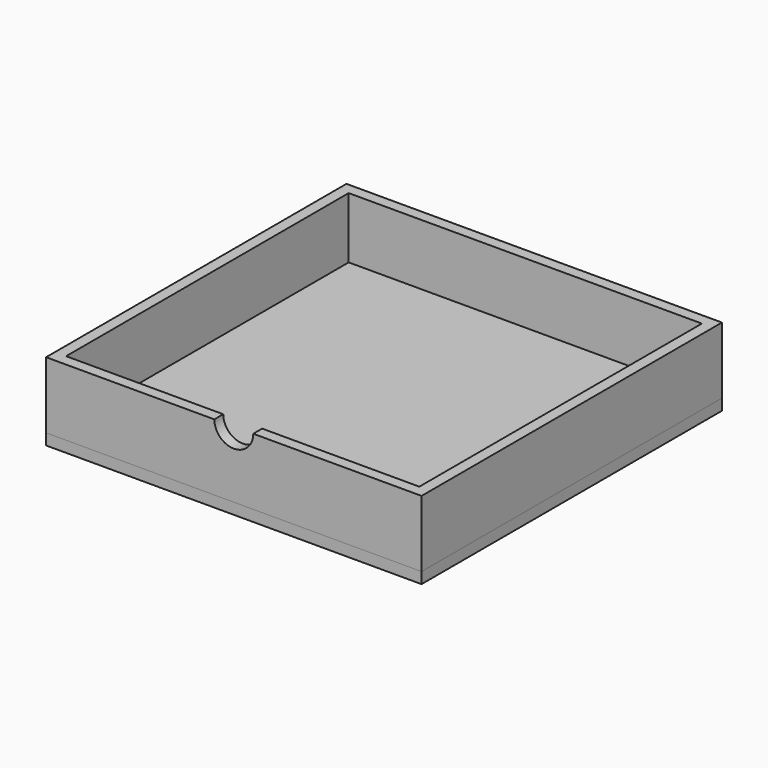
from build123d import *

# Parameters (mm, degrees)
F0_W     = 67.5
F0_H     = 67.5
F0_W_2   = 63.5
F0_H_2   = 63.5
F0_R     = 3.5
F1_DEPTH = 3
F2_DEPTH = 13.97
F4_DEPTH = 2
F5_DEPTH = 2
F6_DEPTH = 3


with BuildPart() as f1:
    # F0 (on Top) → F1 (new body)
    with BuildSketch(Plane.XY):
        Rectangle(F0_W, F0_H)
        Rectangle(F0_W_2, F0_H_2, mode=Mode.SUBTRACT)
        Rectangle(F0_W_2, F0_H_2)
        Circle(F0_R, mode=Mode.SUBTRACT)
    extrude(amount=F1_DEPTH)

    # F0 (on Top) → F2 (join)
    with BuildSketch(Plane.XY):
        Rectangle(F0_W, F0_H)
        Rectangle(F0_W_2, F0_H_2, mode=Mode.SUBTRACT)
    extrude(amount=F2_DEPTH)

    # F3 (on face) → F4 (cut, through all)
    with BuildSketch(Plane.XZ.offset(33.75)):
        with BuildLine():
            ThreePointArc((-3.5, 13.97), (0, 10.47), (3.5, 13.97))
            Line((3.5, 13.97), (-3.5, 13.97))
        make_face()
        with BuildLine():
            Line((-3.5, 13.97), (3.5, 13.97))
            ThreePointArc((3.5, 13.97), (0, 17.47), (-3.5, 13.97))
        make_face()
    extrude(amount=-F4_DEPTH, mode=Mode.SUBTRACT)


with BuildPart() as f5:
    # F0 (on Top) → F5 (new body)
    with BuildSketch(Plane.XY):
        Rectangle(F0_W, F0_H)
        Rectangle(F0_W_2, F0_H_2, mode=Mode.SUBTRACT)
        Rectangle(F0_W_2, F0_H_2)
        Circle(F0_R, mode=Mode.SUBTRACT)
        Circle(F0_R)
    extrude(amount=F5_DEPTH)

    # F0 (on Top) → F6 (join)
    with BuildSketch(Plane.XY):
        Rectangle(F0_W_2, F0_H_2)
        Circle(F0_R, mode=Mode.SUBTRACT)
        Circle(F0_R)
    extrude(amount=F6_DEPTH)


solid = Compound([f1.part, f5.part])
